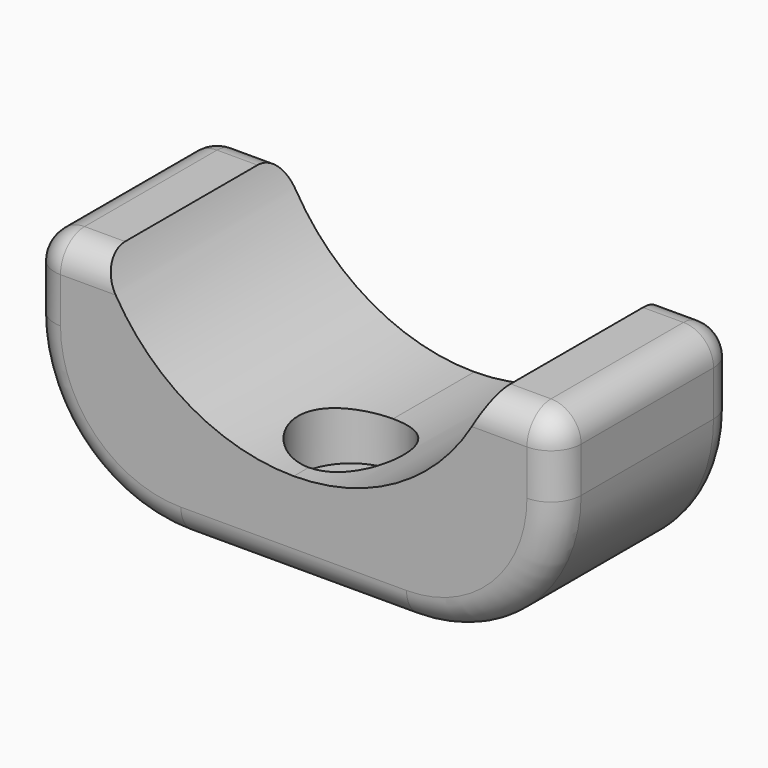
from build123d import *

# Parameters (mm, degrees)
F0_W      = 88.9
F0_H      = 50.8
F1_DEPTH  = 38.1
F3_DEPTH  = 38.101
F5_DEPTH  = 25.4
F7_R      = 8.89
F8_DEPTH  = 25.4
F9_W      = 12.7052063286
F9_H      = 2.550378209
F10_DEPTH = 207.518
F11_F1_R  = 25.4
F11_F2_R  = 25.4
F12_W     = 88.9
F12_H     = 12.7
F13_DEPTH = 56.642
F14_R     = 5.08
F15_DEPTH = 1.27


with BuildPart() as f1:
    # F0 (on Front) → F1 (new body)
    with BuildSketch(Plane.XZ):
        with Locations((44.45, 25.4)):
            Rectangle(F0_W, F0_H)
    extrude(amount=F1_DEPTH)

    # F2 (on face) → F3 (cut, through all)
    with BuildSketch(Plane.XZ.offset(38.1)):
        with BuildLine():
            ThreePointArc((9.525, 50.8), (19.7542956671, 26.1042956671), (44.45, 15.875))
            Line((44.45, 15.875), (44.45, 50.8))
            Line((44.45, 50.8), (9.525, 50.8))
        make_face()
        with BuildLine():
            Line((44.45, 50.8), (44.45, 15.875))
            ThreePointArc((44.45, 15.875), (69.1457043329, 26.1042956671), (79.375, 50.8))
            Line((79.375, 50.8), (44.45, 50.8))
        make_face()
    extrude(amount=-F3_DEPTH, mode=Mode.SUBTRACT)

    # F4 (on face) → F5 (cut)
    with BuildSketch(Plane(origin=(0, 0, 0), x_dir=(1, 0, 0), z_dir=(0, 0, -1))):
        with BuildLine():
            ThreePointArc((47.8282, 26.035), (46.8387481282, 28.4237481282), (44.45, 29.4132))
            ThreePointArc((44.45, 29.4132), (42.0612518718, 23.6462518718), (47.8282, 26.035))
        make_face()
    extrude(amount=-F5_DEPTH, mode=Mode.SUBTRACT)

    # F7 (on offset) → F8 (cut)
    with BuildSketch(Plane.XY.offset(9.525)):
        with Locations((44.45, -26.035)):
            Circle(F7_R)
    extrude(amount=F8_DEPTH, mode=Mode.SUBTRACT)

    # F9 (on face) → F10 (cut)
    with BuildSketch(Plane.YZ.offset(88.9)):
        with Locations((-12.7026031643, 1.2751891045)):
            Rectangle(F9_W, F9_H)
    extrude(amount=-F10_DEPTH, mode=Mode.SUBTRACT)

    # F11: fillet of radius 25.4 on 4 edges, made by hand

    # F11_f1
    f11_f1_edges = [f1.edges().sort_by_distance(p)[0] for p in [
        (0, -3.175, 0),
    ]]
    fillet(f11_f1_edges, radius=F11_F1_R)

    # F11_f2
    f11_f2_edges = [f1.edges().sort_by_distance(p)[0] for p in [
        (88.9, -3.175, 0),
    ]]
    fillet(f11_f2_edges, radius=F11_F2_R)

    # F12 (on face) → F13 (cut)
    with BuildSketch(Plane(origin=(0, 0, 0), x_dir=(-1, 0, 0), z_dir=(0, 1, 0))):
        with Locations((-44.45, 44.45)):
            Rectangle(F12_W, F12_H)
    extrude(amount=-F13_DEPTH, mode=Mode.SUBTRACT)

    # F14
    f14_edges = [f1.edges().sort_by_distance(p)[0] for p in [
        (0, -19.05, 38.1),
        (88.9, -19.05, 38.1),
        (7.439488, -38.1, 7.439488),
        (7.439488, 0, 7.439488),
        (5.957966, -38.1, 38.1),
        (82.942034, -38.1, 38.1),
        (5.957966, 0, 38.1),
        (82.942034, 0, 38.1),
    ]]
    fillet(f14_edges, radius=F14_R)

    # F15 (cut): a face of the model
    f15_faces = [f1.faces().sort_by_distance(p)[0] for p in [
        (35.8114471714, -26.035, 9.525),
    ]]
    extrude(f15_faces, amount=-F15_DEPTH, mode=Mode.SUBTRACT)


solid = f1.part
